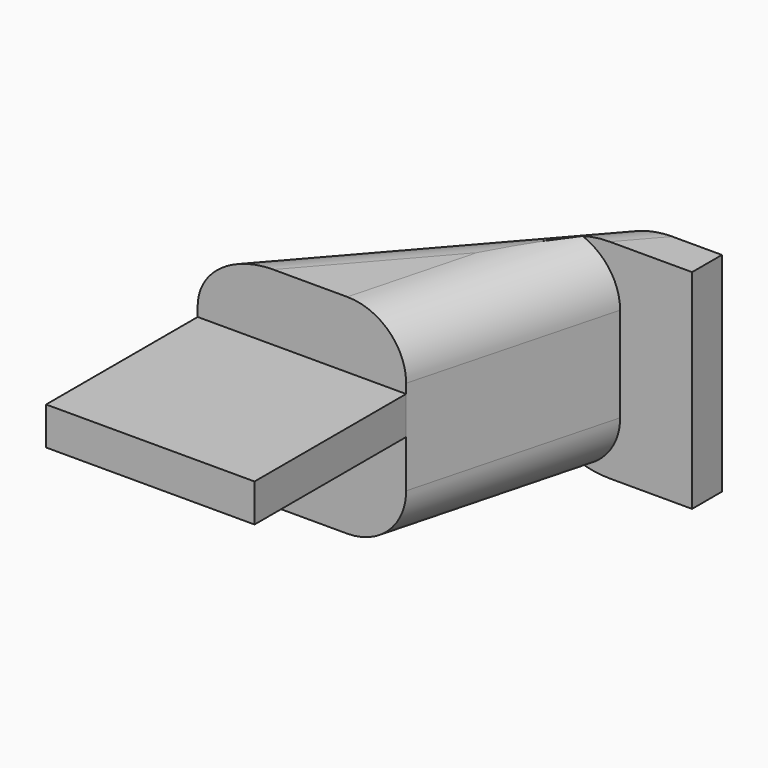
from build123d import *

# Parameters (mm, degrees)
F0_W         = 22
F0_H         = 20
F1_DEPTH     = 4
F2_DEPTH     = 11
F3_DEPTH     = 11
F4_T1_DEPTH  = 63.4073519566
F4_T6_DEPTH  = 51.9365723987
F4_T11_DEPTH = 51.9365723987


# Not quite as in the source:
# - a fillet or chamfer that OpenCascade refuses, or shapes differently, is made with other operations: its cross-section is extruded or revolved along the edge and cut away or added


with BuildPart() as f1:
    # F0 (on Top) → F1 (new body)
    with BuildSketch(Plane.XY):
        with Locations((-11, 10)):
            Rectangle(F0_W, F0_H)
    extrude(amount=F1_DEPTH)

    # F0 (on Top) → F2 (join)
    with BuildSketch(Plane.XY):
        Polygon((-22, 20), (0, 20), (5.6250016205, 41.2031263113), (13.2187530398, 41.2031263113), (13.2187530398, 45.1406277716), (0, 45.1406277716), align=None)
    extrude(amount=F2_DEPTH)

    # F0 (on Top) → F3 (join)
    with BuildSketch(Plane.XY):
        Polygon((-22, 20), (0, 20), (5.6250016205, 41.2031263113), (13.2187530398, 41.2031263113), (13.2187530398, 45.1406277716), (0, 45.1406277716), align=None)
    extrude(amount=-F3_DEPTH)

    # F4: fillet of radius 6 on 4 edges, made by hand

    # F4_s2 → F4_t1 (cut)
    with BuildSketch(Plane(origin=(32.2489050023, 36.8526234865, 0), x_dir=(0, 0, 1), z_dir=(-0.6585376784, -0.7525477567, 0))):
        with BuildLine():
            ThreePointArc((-5, 29.7268042156), (-9.2426406871, 27.9694449027), (-11, 23.7268042156))
            Line((-11, 23.7268042156), (-11, 29.7268042156))
            Line((-11, 29.7268042156), (-5, 29.7268042156))
        make_face()
        with BuildLine():
            ThreePointArc((5, 29.7268042156), (9.2426406871, 27.9694449027), (11, 23.7268042156))
            Line((11, 23.7268042156), (11, 29.7268042156))
            Line((11, 29.7268042156), (5, 29.7268042156))
        make_face()
    extrude(amount=F4_T1_DEPTH, mode=Mode.SUBTRACT)


with BuildPart() as f4_tool4:
    # F4_s5 → F4_t6 (new body)
    with BuildSketch(Plane(origin=(1.1106377761, 4.1864864479, 0), x_dir=(0, 0, 1), z_dir=(0.2564211727, 0.9665651464, 0))):
        with BuildLine():
            ThreePointArc((-11, -11.1284234549), (-9.2426406871, -6.8857827678), (-5, -5.1284234549))
            Line((-5, -5.1284234549), (-11, -5.1284234549))
            Line((-11, -5.1284234549), (-11, -11.1284234549))
        make_face()
    extrude(amount=F4_T6_DEPTH)

    split(bisect_by=Plane.XZ.offset(-41.2031263113), keep=Keep.TOP)


with BuildPart() as f1_1:
    add(f1.part)

    # F4_t3: cut F4_tool4
    add(f4_tool4.part, mode=Mode.SUBTRACT)


with BuildPart() as f4_tool9:
    # F4_s10 → F4_t11 (new body)
    with BuildSketch(Plane(origin=(1.1106377761, 4.1864864479, 0), x_dir=(0, 0, 1), z_dir=(0.2564211727, 0.9665651464, 0))):
        with BuildLine():
            ThreePointArc((11, -11.1284234549), (9.2426406871, -6.8857827678), (5, -5.1284234549))
            Line((5, -5.1284234549), (11, -5.1284234549))
            Line((11, -5.1284234549), (11, -11.1284234549))
        make_face()
    extrude(amount=F4_T11_DEPTH)

    split(bisect_by=Plane.XZ.offset(-41.2031263113), keep=Keep.TOP)


with BuildPart() as f1_2:
    add(f1_1.part)

    # F4_t8: cut F4_tool9
    add(f4_tool9.part, mode=Mode.SUBTRACT)


solid = f1_2.part
